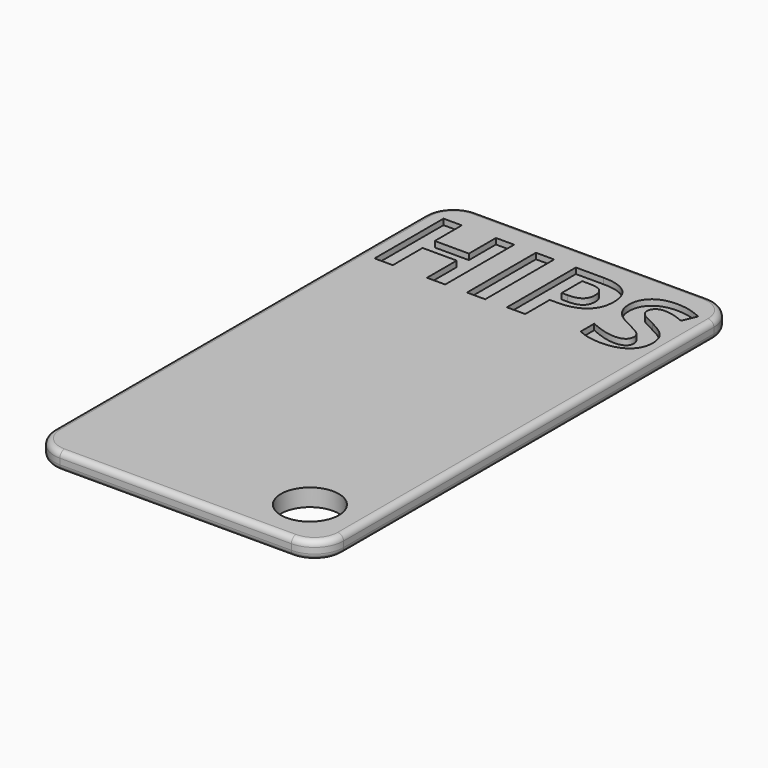
from build123d import *

# Parameters (mm, degrees)
F0_W         = 90
F0_H         = 50
F1_DEPTH     = 3
F2_R         = 1
F3_T1_DEPTH  = 3
F3_T4_ANGLE  = 90
F3_T6_ANGLE  = 90
F3_T8_ANGLE  = 90
F3_T10_ANGLE = 90
F3_T12_ANGLE = 90
F3_T14_ANGLE = 90
F3_T16_ANGLE = 90
F3_T18_ANGLE = 90
F5_ANGLE     = 90
F6_TEXT_SIZE = 20.8667300639
F7_DEPTH     = 1
F8_R         = 5
F9_DEPTH     = 3


# Not quite as in the source:
# - a fillet or chamfer that OpenCascade refuses, or shapes differently, is made with other operations: its cross-section is extruded or revolved along the edge and cut away or added
# - Text() gives the source's letters only with a copy of the font that has no kerning and outlines rounded to 1/6400 em; it was checked with that copy


with BuildPart() as f1:
    # F0 (on Top) → F1 (new body)
    with BuildSketch(Plane.XY):
        Rectangle(F0_W, F0_H)
    extrude(amount=F1_DEPTH)

    # F2
    f2_edges = [f1.edges().sort_by_distance(p)[0] for p in [
        (0, 25, 3),
        (-45, 0, 3),
        (0, -25, 3),
        (45, 0, 3),
        (0, 25, 0),
        (-45, 0, 0),
        (0, -25, 0),
        (45, 0, 0),
    ]]
    fillet(f2_edges, radius=F2_R)

    # F3: fillet of radius 5 on 4 edges, made by hand

    # F3_s2 → F3_t1 (cut)
    with BuildSketch(Plane.XY):
        with BuildLine():
            ThreePointArc((45, -20), (43.5355339059, -23.5355339059), (40, -25))
            Line((40, -25), (45, -25))
            Line((45, -25), (45, -20))
        make_face()
        with BuildLine():
            ThreePointArc((40, 25), (43.5355339059, 23.5355339059), (45, 20))
            Line((45, 20), (45, 25))
            Line((45, 25), (40, 25))
        make_face()
        with BuildLine():
            ThreePointArc((-40, 25), (-43.5355339059, 23.5355339059), (-45, 20))
            Line((-45, 20), (-45, 25))
            Line((-45, 25), (-40, 25))
        make_face()
        with BuildLine():
            ThreePointArc((-45, -20), (-43.5355339059, -23.5355339059), (-40, -25))
            Line((-40, -25), (-45, -25))
            Line((-45, -25), (-45, -20))
        make_face()
    extrude(amount=F3_T1_DEPTH, mode=Mode.SUBTRACT)

    # F3_s3 → F3_t4 (revolve, cut)
    with BuildSketch(Plane.YZ.offset(-40)):
        with BuildLine():
            ThreePointArc((-24, 0), (-24.7071067812, 0.2928932188), (-25, 1))
            Line((-25, 1), (-25, 0))
            Line((-25, 0), (-24, 0))
        make_face()
    revolve(axis=Axis((-40, -20, 0), (0, 0, -1)), revolution_arc=F3_T4_ANGLE, mode=Mode.SUBTRACT)

    # F3_s5 → F3_t6 (revolve, cut)
    with BuildSketch(Plane.XZ.offset(20)):
        with BuildLine():
            ThreePointArc((-44, 3), (-44.7071067812, 2.7071067812), (-45, 2))
            Line((-45, 2), (-45, 3))
            Line((-45, 3), (-44, 3))
        make_face()
    revolve(axis=Axis((-40, -20, 3), (0, 0, 1)), revolution_arc=F3_T6_ANGLE, mode=Mode.SUBTRACT)

    # F3_s7 → F3_t8 (revolve, cut)
    with BuildSketch(Plane.XZ.offset(-20)):
        with BuildLine():
            ThreePointArc((-44, 0), (-44.7071067812, 0.2928932188), (-45, 1))
            Line((-45, 1), (-45, 0))
            Line((-45, 0), (-44, 0))
        make_face()
    revolve(axis=Axis((-40, 20, 0), (0, 0, -1)), revolution_arc=F3_T8_ANGLE, mode=Mode.SUBTRACT)

    # F3_s9 → F3_t10 (revolve, cut)
    with BuildSketch(Plane.YZ.offset(-40)):
        with BuildLine():
            ThreePointArc((24, 3), (24.7071067812, 2.7071067812), (25, 2))
            Line((25, 2), (25, 3))
            Line((25, 3), (24, 3))
        make_face()
    revolve(axis=Axis((-40, 20, 3), (0, 0, 1)), revolution_arc=F3_T10_ANGLE, mode=Mode.SUBTRACT)

    # F3_s11 → F3_t12 (revolve, cut)
    with BuildSketch(Plane.YZ.offset(40)):
        with BuildLine():
            ThreePointArc((24, 0), (24.7071067812, 0.2928932188), (25, 1))
            Line((25, 1), (25, 0))
            Line((25, 0), (24, 0))
        make_face()
    revolve(axis=Axis((40, 20, 0), (0, 0, -1)), revolution_arc=F3_T12_ANGLE, mode=Mode.SUBTRACT)

    # F3_s13 → F3_t14 (revolve, cut)
    with BuildSketch(Plane.XZ.offset(-20)):
        with BuildLine():
            ThreePointArc((44, 3), (44.7071067812, 2.7071067812), (45, 2))
            Line((45, 2), (45, 3))
            Line((45, 3), (44, 3))
        make_face()
    revolve(axis=Axis((40, 20, 3), (0, 0, 1)), revolution_arc=F3_T14_ANGLE, mode=Mode.SUBTRACT)

    # F3_s15 → F3_t16 (revolve, cut)
    with BuildSketch(Plane.XZ.offset(20)):
        with BuildLine():
            ThreePointArc((44, 0), (44.7071067812, 0.2928932188), (45, 1))
            Line((45, 1), (45, 0))
            Line((45, 0), (44, 0))
        make_face()
    revolve(axis=Axis((40, -20, 0), (0, 0, -1)), revolution_arc=F3_T16_ANGLE, mode=Mode.SUBTRACT)

    # F3_s17 → F3_t18 (revolve, cut)
    with BuildSketch(Plane.YZ.offset(40)):
        with BuildLine():
            ThreePointArc((-24, 3), (-24.7071067812, 2.7071067812), (-25, 2))
            Line((-25, 2), (-25, 3))
            Line((-25, 3), (-24, 3))
        make_face()
    revolve(axis=Axis((40, -20, 3), (0, 0, 1)), revolution_arc=F3_T18_ANGLE, mode=Mode.SUBTRACT)


with BuildPart() as f1_1:
    # F5: moved
    add(f1.part.rotate(Axis((0, 0, 16.4477843791), (0, 0, 1)), F5_ANGLE))

    # F6 (on face) → F7 (cut)
    with BuildSketch(Plane.XY.offset(3)):
        with Locations((-24, 25.6153052748)):
            Text('HIPS', F6_TEXT_SIZE, font='Open Sans', font_style=FontStyle.BOLD, text_align=(TextAlign.LEFT, TextAlign.BOTTOM))
    extrude(amount=-F7_DEPTH, mode=Mode.SUBTRACT)

    # F8 (on face) → F9 (cut)
    with BuildSketch(Plane.XY.offset(3)):
        with Locations((16, -36)):
            Circle(F8_R)
    extrude(amount=-F9_DEPTH, mode=Mode.SUBTRACT)


solid = f1_1.part
